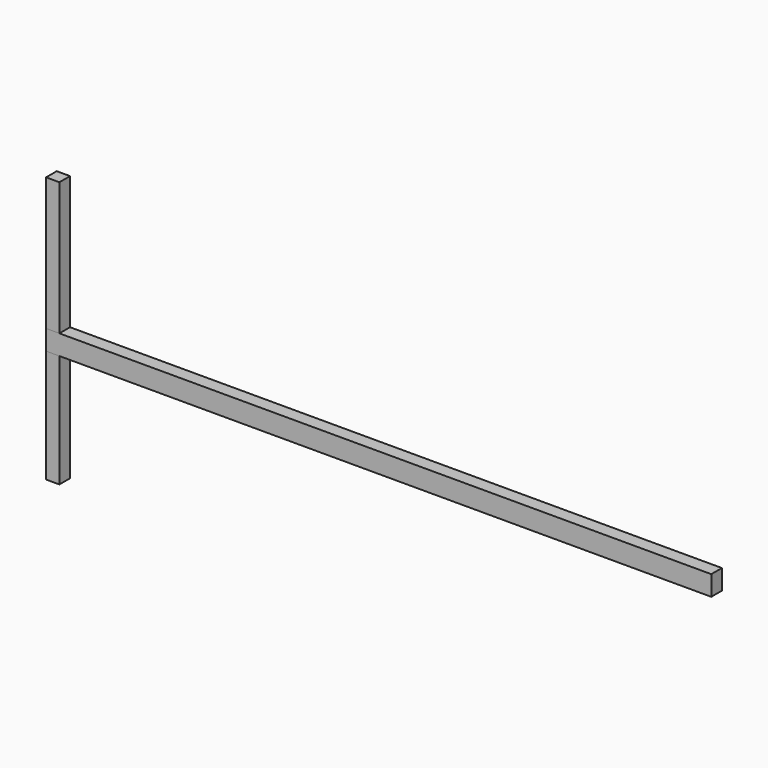
from build123d import *

# Parameters (mm, degrees)
F0_W     = 20
F0_H     = 30
F0_H_2   = 170
F1_DEPTH = 20
F2_DEPTH = 20


# Not quite as in the source:
# - a feature names something its author has since deleted; it is built from what else it names


with BuildPart() as f1:
    # F0 (on Front) → F1 (new body)
    with BuildSketch(Plane.XZ):
        with Locations((-490, 385)):
            Rectangle(F0_W, F0_H)
        Polygon((-480, 370), (-500, 370), (-500, 200), (-480, 200), (-480, 355), align=None)
        with Locations((-490, 85)):
            Rectangle(F0_W, F0_H_2)
        with Locations((-490, 185)):
            Rectangle(F0_W, F0_H)
    extrude(amount=-F1_DEPTH)


with BuildPart() as f2:
    # F0 (on Front) → F2 (new body)
    with BuildSketch(Plane.XZ):
        Polygon((0, 200), (-480, 200), (-480, 170), (0, 170), (480, 170), (480, 200), align=None)
        with Locations((-490, 185)):
            Rectangle(F0_W, F0_H)
        with Locations((490, 185)):
            Rectangle(F0_W, F0_H)
    extrude(amount=-F2_DEPTH)


solid = Compound([f1.part, f2.part])
